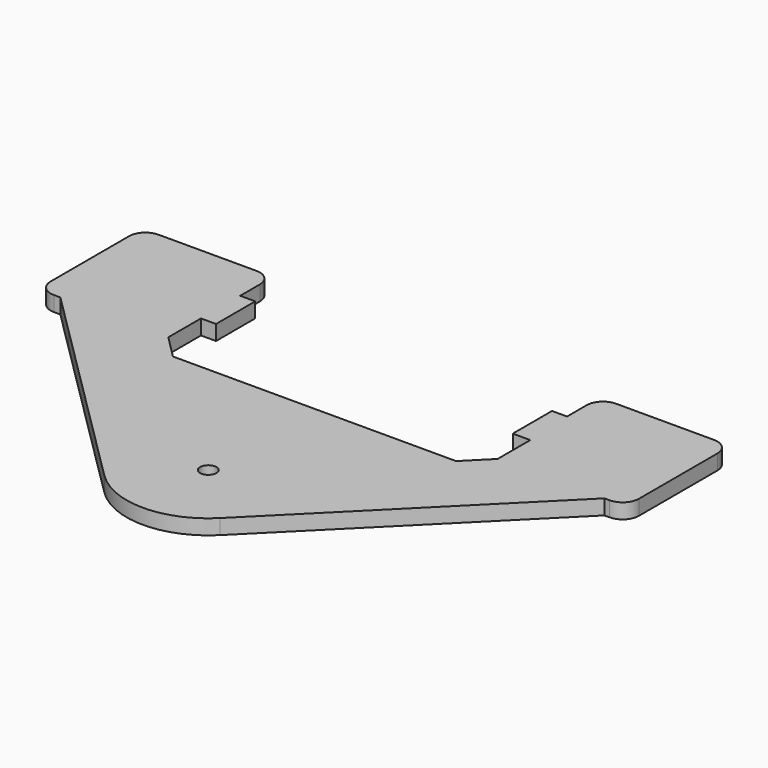
from build123d import *

# Parameters (mm, degrees)
F1_DEPTH = 5.842
F2_R     = 3.175
F3_DEPTH = 5.842


# Not quite as in the source:
# - a feature names something its author has since deleted; it is built from what else it names


with BuildPart() as f1:
    # F0 (on Top) → F1 (new body)
    with BuildSketch(Plane.XY):
        with BuildLine():
            Line((-37.108954253, 15.875), (-43.458954253, 15.875))
            Line((-43.458954253, 15.875), (-75.208954253, 15.875))
            ThreePointArc((-75.208954253, 15.875), (-79.6990823135, 14.0151280605), (-81.558954253, 9.525))
            Line((-81.558954253, 9.525), (-81.558954253, -28.575))
            ThreePointArc((-81.558954253, -28.575), (-79.6990823135, -33.0651280605), (-75.208954253, -34.925))
            Line((-75.208954253, -34.925), (-72.710875161, -34.925))
            Line((-72.710875161, -34.925), (-56.7378558105, -50.8045013442))
            Line((-56.7378558105, -50.8045013442), (10.8431089825, -117.9897966054))
            ThreePointArc((10.8431089825, -117.9897966054), (21.0344920397, -66.1580316621), (64.9777384297, -95.4733389685))
            ThreePointArc((64.9777384297, -95.4733389685), (62.5609135869, -107.6235379461), (55.6783787323, -117.9239792712))
            Line((55.6783787323, -117.9239792712), (110.9403548131, -62.6620031905))
            Line((110.9403548131, -62.6620031905), (138.6796593377, -34.9226986659))
            Line((138.6796593377, -34.9226986659), (140.691045747, -34.9226986659))
            ThreePointArc((140.691045747, -34.9226986659), (145.1811738076, -33.0628267264), (147.041045747, -28.5726986659))
            Line((147.041045747, -28.5726986659), (147.041045747, 9.525))
            ThreePointArc((147.041045747, 9.525), (145.1811738076, 14.0151280605), (140.691045747, 15.875))
            Line((140.691045747, 15.875), (108.941045747, 15.875))
            Line((108.941045747, 15.875), (102.591045747, 15.875))
            ThreePointArc((102.591045747, 15.875), (98.1009176865, 14.0151280605), (96.241045747, 9.525))
            Line((96.241045747, 9.525), (96.241045747, 0))
            Line((96.241045747, 0), (90.399045747, 0))
            Line((90.399045747, 0), (90.399045747, -19.05))
            Line((90.399045747, -19.05), (97.2144311123, -19.05))
            Line((97.2144311123, -19.05), (97.2144311123, -34.925))
            Line((97.2144311123, -34.925), (88.2341749912, -43.9052561211))
            Line((88.2341749912, -43.9052561211), (-21.7786981319, -43.9052561211))
            Line((-21.7786981319, -43.9052561211), (-30.758954253, -34.925))
            Line((-30.758954253, -34.925), (-30.758954253, -19.05))
            Line((-30.758954253, -19.05), (-24.916954253, -19.05))
            Line((-24.916954253, -19.05), (-24.916954253, 0))
            Line((-24.916954253, 0), (-30.758954253, 0))
            Line((-30.758954253, 0), (-30.758954253, 9.525))
            ThreePointArc((-30.758954253, 9.525), (-32.6188261924, 14.0151280605), (-37.108954253, 15.875))
        make_face()
        with BuildLine():
            ThreePointArc((64.9777384297, -95.4733389685), (21.0344920397, -66.1580316621), (10.8431089825, -117.9897966054))
            ThreePointArc((10.8431089825, -117.9897966054), (33.2743467834, -127.2233047585), (55.6783787323, -117.9239792712))
            ThreePointArc((55.6783787323, -117.9239792712), (62.5609135869, -107.6235379461), (64.9777384297, -95.4733389685))
        make_face()
    extrude(amount=F1_DEPTH)

    # F2 (on face) → F3 (cut, through all)
    with BuildSketch(Plane.XY.offset(5.842)):
        with Locations((33.2277384297, -95.4733389685)):
            Circle(F2_R)
    extrude(amount=-F3_DEPTH, mode=Mode.SUBTRACT)


solid = f1.part
